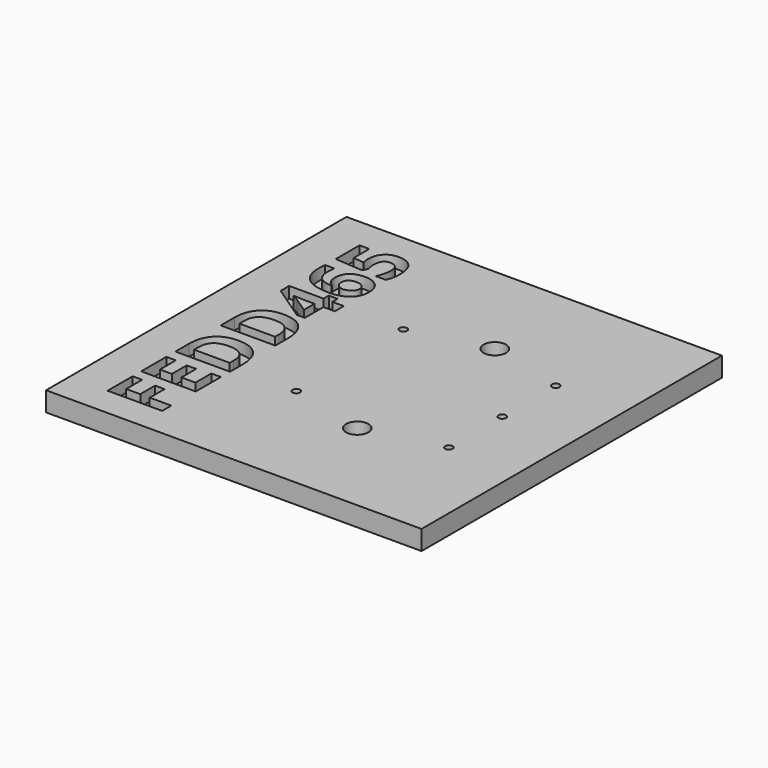
from build123d import *

# Parameters (mm, degrees)
F0_W         = 50
F0_H         = 50
F1_DEPTH     = 2.6
F2_TEXT_SIZE = 10.1807664497
F3_DEPTH     = 1.5
F4_R         = 0.5
F4_R_2       = 1.5
F5_DEPTH     = 2.6


# Not quite as in the source:
# - Text() gives the source's letters only with a copy of the font that has no kerning and outlines rounded to 1/6400 em; it was checked with that copy


with BuildPart() as f1:
    # F0 (on Top) → F1 (new body)
    with BuildSketch(Plane.XY):
        with Locations((-18.1587231159, 3.3350909071)):
            Rectangle(F0_W, F0_H)
    extrude(amount=F1_DEPTH)

    # F2 (on face) → F3 (cut)
    with BuildSketch(Plane.XY.offset(2.6)):
        with Locations(Location((-30.8285712721, -18.6649090929), (0, 0, 90))):
            Text('FEDD465', F2_TEXT_SIZE, font='Open Sans', font_style=FontStyle.BOLD, text_align=(TextAlign.LEFT, TextAlign.BOTTOM))
    extrude(amount=-F3_DEPTH, mode=Mode.SUBTRACT)

    # F4 (on face) → F5 (cut, through all)
    with BuildSketch(Plane.XY.offset(2.6)):
        with Locations((-22.7087231159, -5.5649090929)):
            Circle(F4_R)
        with Locations((-12.5587231159, 14.7850909071)):
            Circle(F4_R_2)
        with Locations((-12.5587231159, -8.1149090929)):
            Circle(F4_R_2)
        with Locations((-22.7087231159, 12.2350909071)):
            Circle(F4_R)
        with Locations((-2.4087231159, -5.5649090929)):
            Circle(F4_R)
        with Locations((-2.4087231159, 3.3350909071)):
            Circle(F4_R)
        with Locations((-2.4087231159, 12.2350909071)):
            Circle(F4_R)
    extrude(amount=-F5_DEPTH, mode=Mode.SUBTRACT)


solid = f1.part
